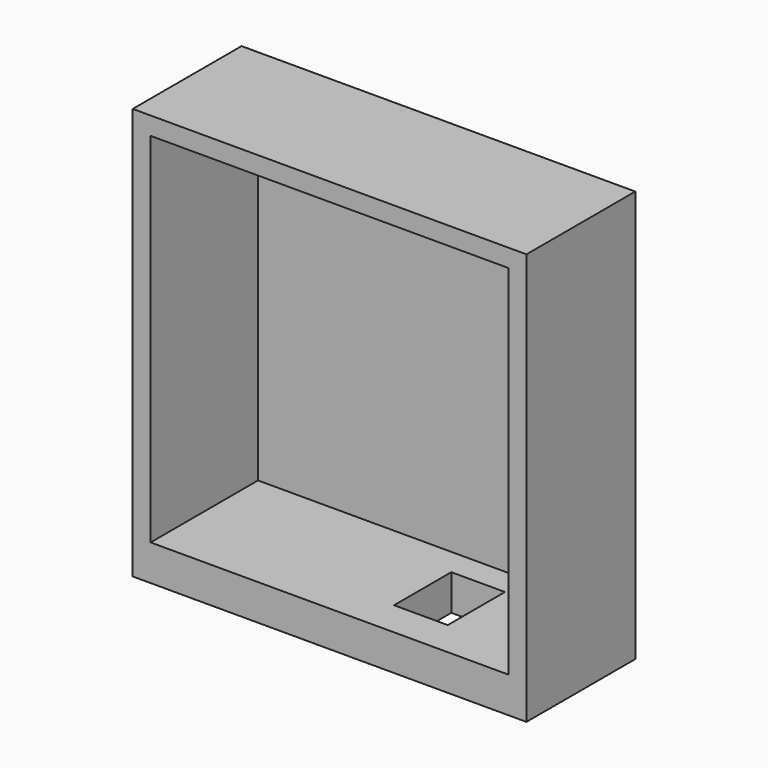
from build123d import *

# Parameters (mm, degrees)
F0_W     = 6705.6
F0_H     = 7010.4
F0_W_2   = 6096
F0_H_2   = 6096
F1_DEPTH = 2316.48
F2_DEPTH = 30.48
F5_W     = 914.4
F5_H     = 1219.2
F6_DEPTH = 609.6


# Not quite as in the source:
# - the program builds the solid bodies; features that only make, move or delete a surface that nothing else refers to are left out


with BuildPart() as f1:
    # F0 (on Front) → F1 (new body)
    with BuildSketch(Plane.XZ):
        with Locations((0, -152.4)):
            Rectangle(F0_W, F0_H)
        Rectangle(F0_W_2, F0_H_2, mode=Mode.SUBTRACT)
    extrude(amount=F1_DEPTH)

    # F0 (on Front) → F2 (join)
    with BuildSketch(Plane.XZ):
        Rectangle(F0_W_2, F0_H_2)
    extrude(amount=F2_DEPTH)

    # F5 (on face) → F6 (cut, through all)
    with BuildSketch(Plane(origin=(0, 0, -3657.6), x_dir=(1, 0, 0), z_dir=(0, 0, -1))):
        with Locations((1066.8, 1097.28)):
            Rectangle(F5_W, F5_H)
    extrude(amount=-F6_DEPTH, mode=Mode.SUBTRACT)


solid = f1.part
